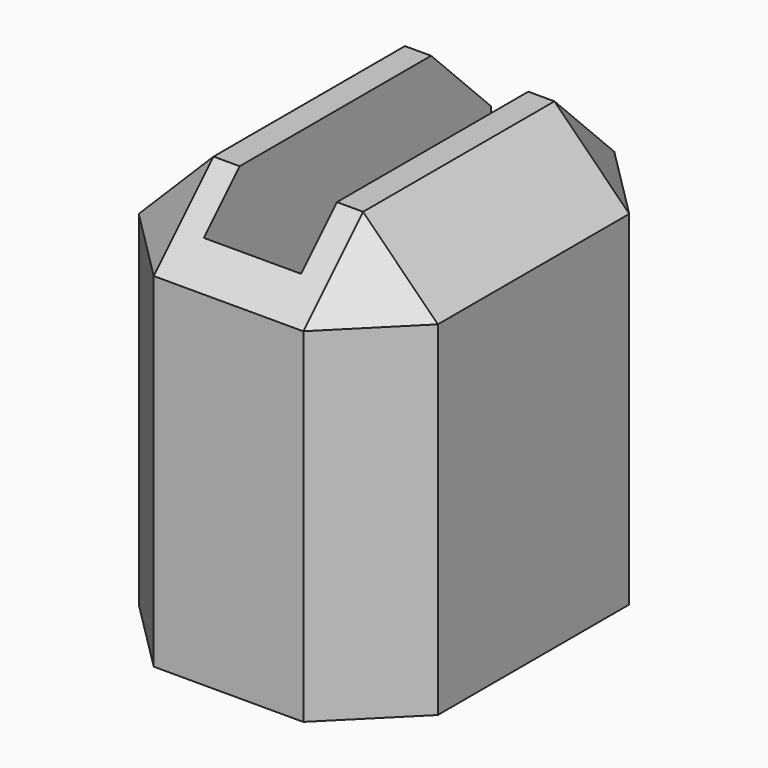
from build123d import *

# Parameters (mm, degrees)
F0_W          = 20
F0_H          = 26
F1_DEPTH      = 28
F3_DEPTH      = 3.25
F3_DEPTH_BACK = 3.25
F4_T1_DEPTH   = 6.3508529611
F4_T3_DEPTH   = 6.3508529611
F4_T5_DEPTH   = 6.3508529611
F4_T7_DEPTH   = 6.3508529611
F4_T9_DEPTH   = 51.7168298797
F4_T11_DEPTH  = 45.7168298797
F4_T13_DEPTH  = 53.7168298797
F4_T15_DEPTH  = 32.4668298797
F4_T17_DEPTH  = 32.4668298797


# Not quite as in the source:
# - a fillet or chamfer that OpenCascade refuses, or shapes differently, is made with other operations: its cross-section is extruded or revolved along the edge and cut away or added


with BuildPart() as f1:
    # F0 (on Top) → F1 (new body)
    with BuildSketch(Plane.XY):
        Rectangle(F0_W, F0_H)
    extrude(amount=F1_DEPTH)

    # F2 (on Right) → F3 (cut, two sides)
    with BuildSketch(Plane.YZ) as f3_sk:
        Polygon((13, 28), (-11, 28), (-11, 19.4068542495), (-5.3431457505, 13.75), (13, 13.75), align=None)
    extrude(amount=-F3_DEPTH, mode=Mode.SUBTRACT)
    extrude(f3_sk.sketch, amount=F3_DEPTH_BACK, mode=Mode.SUBTRACT)

    # F4: chamfer of 5 on 9 edges, made by hand

    # F4_s2 → F4_t1 (cut)
    with BuildSketch(Plane(origin=(13.6666666667, -13.6666666667, 13.6666666667), x_dir=(0.7071067812, 0.7071067812, 0), z_dir=(0.5773502692, -0.5773502692, 0.5773502692))):
        Polygon((1.4142135624, 11.430952133), (-5.6568542495, 11.430952133), (-2.1213203436, 17.5546764899), align=None)
    extrude(amount=F4_T1_DEPTH, mode=Mode.SUBTRACT)

    # F4_s4 → F4_t3 (cut)
    with BuildSketch(Plane(origin=(13.6666666667, 13.6666666667, 13.6666666667), x_dir=(-0.7071067812, 0.7071067812, 0), z_dir=(0.5773502692, 0.5773502692, 0.5773502692))):
        Polygon((-1.4142135624, 11.430952133), (5.6568542495, 11.430952133), (2.1213203436, 17.5546764899), align=None)
    extrude(amount=F4_T3_DEPTH, mode=Mode.SUBTRACT)

    # F4_s6 → F4_t5 (cut)
    with BuildSketch(Plane(origin=(-13.6666666667, -13.6666666667, 13.6666666667), x_dir=(0.7071067812, -0.7071067812, 0), z_dir=(-0.5773502692, -0.5773502692, 0.5773502692))):
        Polygon((5.6568542495, 11.430952133), (2.1213203436, 17.5546764899), (-1.4142135624, 11.430952133), align=None)
    extrude(amount=F4_T5_DEPTH, mode=Mode.SUBTRACT)

    # F4_s8 → F4_t7 (cut)
    with BuildSketch(Plane(origin=(-13.6666666667, 13.6666666667, 13.6666666667), x_dir=(-0.7071067812, -0.7071067812, 0), z_dir=(-0.5773502692, 0.5773502692, 0.5773502692))):
        Polygon((-5.6568542495, 11.430952133), (-2.1213203436, 17.5546764899), (1.4142135624, 11.430952133), align=None)
    extrude(amount=F4_T7_DEPTH, mode=Mode.SUBTRACT)

    # F4_s10 → F4_t9 (cut)
    with BuildSketch(Plane.XZ.offset(-25.8584149398)):
        Polygon((10, 23), (5, 28), (10, 28), align=None)
        Polygon((-5, 28), (-10, 23), (-10, 28), align=None)
    extrude(amount=F4_T9_DEPTH, mode=Mode.SUBTRACT)

    # F4_s12 → F4_t11 (cut)
    with BuildSketch(Plane.YZ.offset(-22.8584149398)):
        Polygon((-13, 23), (-8, 28), (-13, 28), align=None)
    extrude(amount=F4_T11_DEPTH, mode=Mode.SUBTRACT)

    # F4_s14 → F4_t13 (cut)
    with BuildSketch(Plane.XY.offset(-12.8584149398)):
        Polygon((10, -8), (5, -13), (10, -13), align=None)
        Polygon((-5, -13), (-10, -8), (-10, -13), align=None)
        Polygon((10, 8), (5, 13), (10, 13), align=None)
        Polygon((-5, 13), (-10, 8), (-10, 13), align=None)
    extrude(amount=F4_T13_DEPTH, mode=Mode.SUBTRACT)

    # F4_s16 → F4_t15 (cut)
    with BuildSketch(Plane.YZ.offset(-22.8584149398)):
        Polygon((13, 23), (8, 28), (13, 28), align=None)
    extrude(amount=F4_T15_DEPTH, mode=Mode.SUBTRACT)

    # F4_s18 → F4_t17 (cut)
    with BuildSketch(Plane.YZ.offset(-9.6084149398)):
        Polygon((13, 23), (8, 28), (13, 28), align=None)
    extrude(amount=F4_T17_DEPTH, mode=Mode.SUBTRACT)


solid = f1.part
